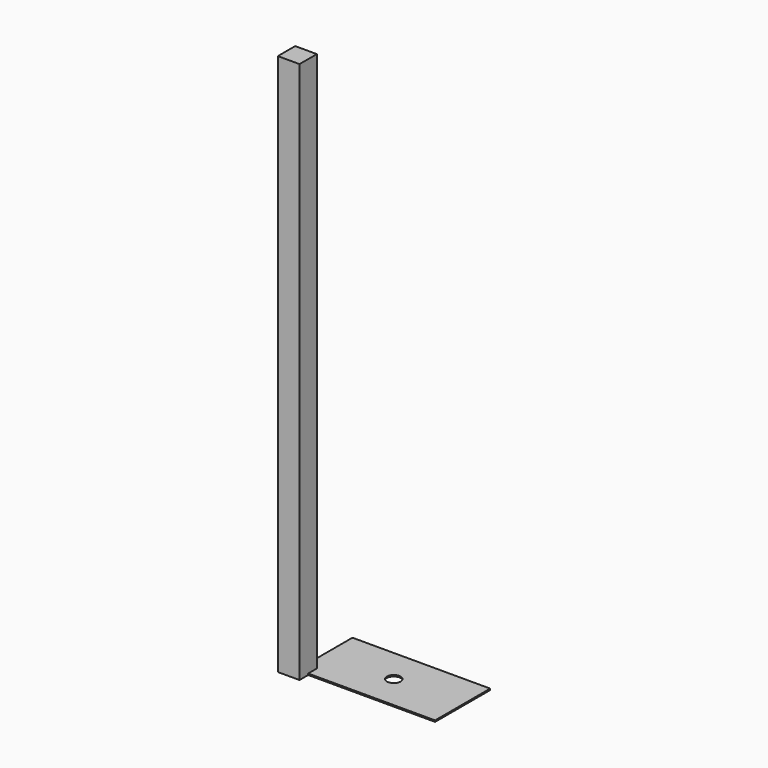
from build123d import *

# Parameters (mm, degrees)
F0_W     = 40
F0_H     = 40
F1_DEPTH = 1000
F2_W     = 254
F2_H     = 127
F2_R     = 12.7
F3_DEPTH = 0.254
F4_DEPTH = 2.54


with BuildPart() as f1:
    # F0 (on Top) → F1 (new body)
    with BuildSketch(Plane.XY):
        Rectangle(F0_W, F0_H)
    extrude(amount=F1_DEPTH)


with BuildPart() as f3:
    # F2 (on Top) → F3 (new body)
    with BuildSketch(Plane.XY):
        with Locations((127, 63.5)):
            Rectangle(F2_W, F2_H)
        with Locations((127, 63.5)):
            Circle(F2_R, mode=Mode.SUBTRACT)
    extrude(amount=F3_DEPTH)

    # F2 (on Top) → F4 (join)
    with BuildSketch(Plane.XY):
        with Locations((127, 63.5)):
            Rectangle(F2_W, F2_H)
        with Locations((127, 63.5)):
            Circle(F2_R, mode=Mode.SUBTRACT)
    extrude(amount=F4_DEPTH)


solid = Compound([f1.part, f3.part])
